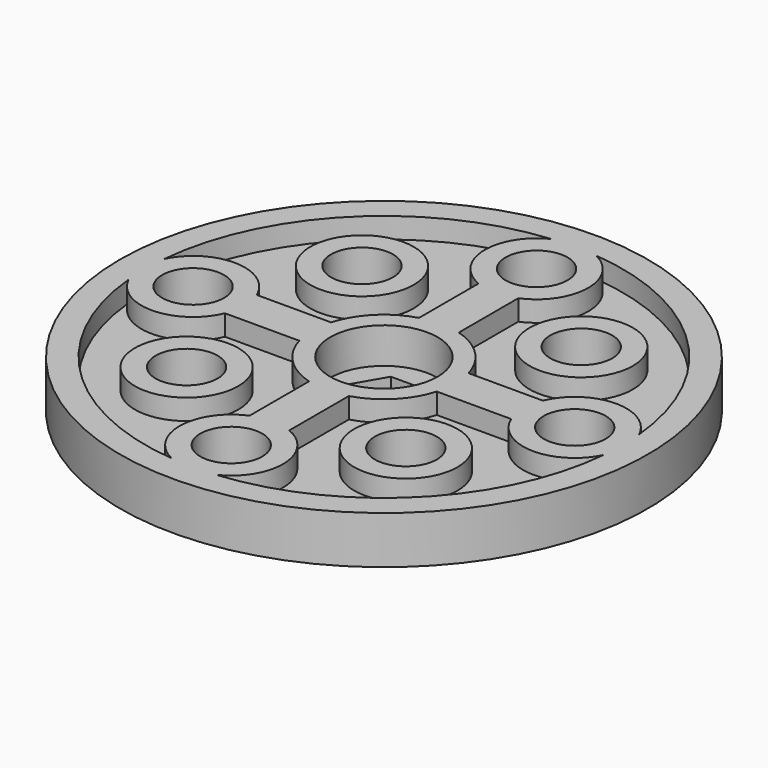
from build123d import *

# Parameters (mm, degrees)
F0_R     = 3.375
F0_R_2   = 1.95
F1_DEPTH = 3
F0_R_3   = 3.25
F2_DEPTH = 1.7
F3_DEPTH = 3
F4_R     = 3.375
F5_DEPTH = 2.25
F6_R     = 4.5310889132
F7_DEPTH = 3.75
F8_R     = 0.75


# Not quite as in the source:
# - a feature names something its author has since deleted; it is built from what else it names


with BuildPart() as f1:
    # F0 (on Top) → F1 (new body)
    with BuildSketch(Plane.XY):
        with BuildLine():
            ThreePointArc((16.6, 0), (0, 16.6), (-16.6, 0))
            ThreePointArc((-16.6, 0), (0, -16.6), (16.6, 0))
        make_face()
        with BuildLine():
            ThreePointArc((14.9348958333, 1.3960252317), (14.9837151184, 0.698771243), (15, 0))
            ThreePointArc((15, 0), (14.9837151184, -0.698771243), (14.9348958333, -1.3960252317))
            ThreePointArc((14.9348958333, -1.3960252317), (10.6066017178, -10.6066017178), (1.3960252317, -14.9348958333))
            ThreePointArc((1.3960252317, -14.9348958333), (0, -15), (-1.3960252317, -14.9348958333))
            ThreePointArc((-1.3960252317, -14.9348958333), (-10.6066017178, -10.6066017178), (-14.9348958333, -1.3960252317))
            ThreePointArc((-14.9348958333, -1.3960252317), (-14.9837151184, -0.698771243), (-15, 0))
            ThreePointArc((-15, 0), (-14.9837151184, 0.698771243), (-14.9348958333, 1.3960252317))
            ThreePointArc((-14.9348958333, 1.3960252317), (-10.6066017178, 10.6066017178), (-1.3960252317, 14.9348958333))
            ThreePointArc((-1.3960252317, 14.9348958333), (0, 15), (1.3960252317, 14.9348958333))
            ThreePointArc((1.3960252317, 14.9348958333), (10.6066017178, 10.6066017178), (14.9348958333, 1.3960252317))
        make_face(mode=Mode.SUBTRACT)
        with BuildLine():
            ThreePointArc((1.25, -4.3229041164), (3.1819805153, -3.1819805153), (4.3229041164, -1.25))
            ThreePointArc((4.3229041164, -1.25), (4.4555060613, -0.6312414261), (4.5, 0))
            ThreePointArc((4.5, 0), (4.4555060613, 0.6312414261), (4.3229041164, 1.25))
            ThreePointArc((4.3229041164, 1.25), (3.1819805153, 3.1819805153), (1.25, 4.3229041164))
            ThreePointArc((1.25, 4.3229041164), (0, 4.5), (-1.25, 4.3229041164))
            ThreePointArc((-1.25, 4.3229041164), (-3.1819805153, 3.1819805153), (-4.3229041164, 1.25))
            ThreePointArc((-4.3229041164, 1.25), (-4.5, 0), (-4.3229041164, -1.25))
            ThreePointArc((-4.3229041164, -1.25), (-3.1819805153, -3.1819805153), (-1.25, -4.3229041164))
            ThreePointArc((-1.25, -4.3229041164), (0, -4.5), (1.25, -4.3229041164))
        make_face()
        Circle(F0_R, mode=Mode.SUBTRACT)
        Circle(F0_R)
        Polygon((-2.25, 0), (-1.125, 1.9485571585), (1.125, 1.9485571585), (2.25, 0), (1.125, -1.9485571585), (-1.125, -1.9485571585), align=None, mode=Mode.SUBTRACT)
        with BuildLine():
            ThreePointArc((14.9348958333, -1.3960252317), (14.9837151184, -0.698771243), (15, 0))
            ThreePointArc((15, 0), (14.9837151184, 0.698771243), (14.9348958333, 1.3960252317))
            ThreePointArc((14.9348958333, 1.3960252317), (11.9200595209, 3.2490167004), (9, 1.25))
            ThreePointArc((9, 1.25), (8.75, 0), (9, -1.25))
            ThreePointArc((9, -1.25), (11.9200595209, -3.2490167004), (14.9348958333, -1.3960252317))
        make_face()
        with Locations((12, 0)):
            Circle(F0_R_2, mode=Mode.SUBTRACT)
        with BuildLine():
            ThreePointArc((1.25, 9), (3.2490167004, 11.9200595209), (1.3960252317, 14.9348958333))
            ThreePointArc((1.3960252317, 14.9348958333), (0, 15), (-1.3960252317, 14.9348958333))
            ThreePointArc((-1.3960252317, 14.9348958333), (-3.2490167004, 11.9200595209), (-1.25, 9))
            ThreePointArc((-1.25, 9), (0, 8.75), (1.25, 9))
        make_face()
        with Locations((0, 12)):
            Circle(F0_R_2, mode=Mode.SUBTRACT)
        with BuildLine():
            ThreePointArc((-1.3960252317, -14.9348958333), (0, -15), (1.3960252317, -14.9348958333))
            ThreePointArc((1.3960252317, -14.9348958333), (3.2490167004, -11.9200595209), (1.25, -9))
            ThreePointArc((1.25, -9), (0, -8.75), (-1.25, -9))
            ThreePointArc((-1.25, -9), (-3.2490167004, -11.9200595209), (-1.3960252317, -14.9348958333))
        make_face()
        with Locations((0, -12)):
            Circle(F0_R_2, mode=Mode.SUBTRACT)
        with BuildLine():
            ThreePointArc((-9, 1.25), (-11.9200595209, 3.2490167004), (-14.9348958333, 1.3960252317))
            ThreePointArc((-14.9348958333, 1.3960252317), (-14.9837151184, 0.698771243), (-15, 0))
            ThreePointArc((-15, 0), (-14.9837151184, -0.698771243), (-14.9348958333, -1.3960252317))
            ThreePointArc((-14.9348958333, -1.3960252317), (-11.9200595209, -3.2490167004), (-9, -1.25))
            ThreePointArc((-9, -1.25), (-8.75, 0), (-9, 1.25))
        make_face()
        with Locations((-12, 0)):
            Circle(F0_R_2, mode=Mode.SUBTRACT)
        with BuildLine():
            ThreePointArc((9, -1.25), (8.75, 0), (9, 1.25))
            Line((9, 1.25), (6, 1.25))
            Line((6, 1.25), (4.3229041164, 1.25))
            ThreePointArc((4.3229041164, 1.25), (4.4555060613, 0.6312414261), (4.5, 0))
            ThreePointArc((4.5, 0), (4.4555060613, -0.6312414261), (4.3229041164, -1.25))
            Line((4.3229041164, -1.25), (9, -1.25))
        make_face()
        with BuildLine():
            Line((1.25, 4.3229041164), (1.25, 9))
            ThreePointArc((1.25, 9), (0, 8.75), (-1.25, 9))
            Line((-1.25, 9), (-1.25, 6))
            Line((-1.25, 6), (-1.25, 4.3229041164))
            ThreePointArc((-1.25, 4.3229041164), (0, 4.5), (1.25, 4.3229041164))
        make_face()
        with BuildLine():
            ThreePointArc((-1.25, -9), (0, -8.75), (1.25, -9))
            Line((1.25, -9), (1.25, -6))
            Line((1.25, -6), (1.25, -4.3229041164))
            ThreePointArc((1.25, -4.3229041164), (0, -4.5), (-1.25, -4.3229041164))
            Line((-1.25, -4.3229041164), (-1.25, -9))
        make_face()
        with BuildLine():
            Line((-4.3229041164, 1.25), (-9, 1.25))
            ThreePointArc((-9, 1.25), (-8.75, 0), (-9, -1.25))
            Line((-9, -1.25), (-6, -1.25))
            Line((-6, -1.25), (-4.3229041164, -1.25))
            ThreePointArc((-4.3229041164, -1.25), (-4.5, 0), (-4.3229041164, 1.25))
        make_face()
    extrude(amount=F1_DEPTH)



with BuildPart() as f1b:
    # F0 (on Top) → F1, piece 2 (new body)
    with BuildSketch(Plane.XY):
        with Locations((6.8942911166, 6.8942911166)):
            Circle(F0_R_3)
        with Locations((6.8942911166, 6.8942911166)):
            Circle(F0_R_2, mode=Mode.SUBTRACT)
    extrude(amount=F1_DEPTH)


with BuildPart() as f1c:
    # F0 (on Top) → F1, piece 3 (new body)
    with BuildSketch(Plane.XY):
        with Locations((-6.8942911166, 6.8942911166)):
            Circle(F0_R_3)
        with Locations((-6.8942911166, 6.8942911166)):
            Circle(F0_R_2, mode=Mode.SUBTRACT)
    extrude(amount=F1_DEPTH)


with BuildPart() as f1d:
    # F0 (on Top) → F1, piece 4 (new body)
    with BuildSketch(Plane.XY):
        with Locations((-6.8942911166, -6.8942911166)):
            Circle(F0_R_3)
        with Locations((-6.8942911166, -6.8942911166)):
            Circle(F0_R_2, mode=Mode.SUBTRACT)
    extrude(amount=F1_DEPTH)


with BuildPart() as f1e:
    # F0 (on Top) → F1, piece 5 (new body)
    with BuildSketch(Plane.XY):
        with Locations((6.8942911166, -6.8942911166)):
            Circle(F0_R_3)
        with Locations((6.8942911166, -6.8942911166)):
            Circle(F0_R_2, mode=Mode.SUBTRACT)
    extrude(amount=F1_DEPTH)


with BuildPart() as f1_1:
    add(f1.part)

    add(f1b.part)  # F2 merges F1b

    add(f1c.part)  # F2 merges F1c

    add(f1d.part)  # F2 merges F1d

    add(f1e.part)  # F2 merges F1e
    # F0 (on Top) → F2 (join)
    with BuildSketch(Plane.XY):
        with BuildLine():
            ThreePointArc((-1.25, 9), (-3.2490167004, 11.9200595209), (-1.3960252317, 14.9348958333))
            ThreePointArc((-1.3960252317, 14.9348958333), (-10.6066017178, 10.6066017178), (-14.9348958333, 1.3960252317))
            ThreePointArc((-14.9348958333, 1.3960252317), (-11.9200595209, 3.2490167004), (-9, 1.25))
            Line((-9, 1.25), (-4.3229041164, 1.25))
            ThreePointArc((-4.3229041164, 1.25), (-3.1819805153, 3.1819805153), (-1.25, 4.3229041164))
            Line((-1.25, 4.3229041164), (-1.25, 6))
            Line((-1.25, 6), (-1.25, 9))
        make_face()
        with Locations((-6.8942911166, 6.8942911166)):
            Circle(F0_R_3, mode=Mode.SUBTRACT)
        with BuildLine():
            ThreePointArc((9, 1.25), (11.9200595209, 3.2490167004), (14.9348958333, 1.3960252317))
            ThreePointArc((14.9348958333, 1.3960252317), (10.6066017178, 10.6066017178), (1.3960252317, 14.9348958333))
            ThreePointArc((1.3960252317, 14.9348958333), (3.2490167004, 11.9200595209), (1.25, 9))
            Line((1.25, 9), (1.25, 4.3229041164))
            ThreePointArc((1.25, 4.3229041164), (3.1819805153, 3.1819805153), (4.3229041164, 1.25))
            Line((4.3229041164, 1.25), (6, 1.25))
            Line((6, 1.25), (9, 1.25))
        make_face()
        with Locations((6.8942911166, 6.8942911166)):
            Circle(F0_R_3, mode=Mode.SUBTRACT)
        with BuildLine():
            ThreePointArc((1.3960252317, -14.9348958333), (10.6066017178, -10.6066017178), (14.9348958333, -1.3960252317))
            ThreePointArc((14.9348958333, -1.3960252317), (11.9200595209, -3.2490167004), (9, -1.25))
            Line((9, -1.25), (4.3229041164, -1.25))
            ThreePointArc((4.3229041164, -1.25), (3.1819805153, -3.1819805153), (1.25, -4.3229041164))
            Line((1.25, -4.3229041164), (1.25, -6))
            Line((1.25, -6), (1.25, -9))
            ThreePointArc((1.25, -9), (3.2490167004, -11.9200595209), (1.3960252317, -14.9348958333))
        make_face()
        with Locations((6.8942911166, -6.8942911166)):
            Circle(F0_R_3, mode=Mode.SUBTRACT)
        with BuildLine():
            ThreePointArc((-14.9348958333, -1.3960252317), (-10.6066017178, -10.6066017178), (-1.3960252317, -14.9348958333))
            ThreePointArc((-1.3960252317, -14.9348958333), (-3.2490167004, -11.9200595209), (-1.25, -9))
            Line((-1.25, -9), (-1.25, -4.3229041164))
            ThreePointArc((-1.25, -4.3229041164), (-3.1819805153, -3.1819805153), (-4.3229041164, -1.25))
            Line((-4.3229041164, -1.25), (-6, -1.25))
            Line((-6, -1.25), (-9, -1.25))
            ThreePointArc((-9, -1.25), (-11.9200595209, -3.2490167004), (-14.9348958333, -1.3960252317))
        make_face()
        with Locations((-6.8942911166, -6.8942911166)):
            Circle(F0_R_3, mode=Mode.SUBTRACT)
        Circle(F0_R)
        Polygon((-2.25, 0), (-1.125, 1.9485571585), (1.125, 1.9485571585), (2.25, 0), (1.125, -1.9485571585), (-1.125, -1.9485571585), align=None, mode=Mode.SUBTRACT)
    extrude(amount=F2_DEPTH)

    # F0 (on Top) → F3 (join)
    with BuildSketch(Plane.XY):
        with BuildLine():
            ThreePointArc((16.6, 0), (0, 16.6), (-16.6, 0))
            ThreePointArc((-16.6, 0), (0, -16.6), (16.6, 0))
        make_face()
        with BuildLine():
            ThreePointArc((14.9348958333, 1.3960252317), (14.9837151184, 0.698771243), (15, 0))
            ThreePointArc((15, 0), (14.9837151184, -0.698771243), (14.9348958333, -1.3960252317))
            ThreePointArc((14.9348958333, -1.3960252317), (10.6066017178, -10.6066017178), (1.3960252317, -14.9348958333))
            ThreePointArc((1.3960252317, -14.9348958333), (0, -15), (-1.3960252317, -14.9348958333))
            ThreePointArc((-1.3960252317, -14.9348958333), (-10.6066017178, -10.6066017178), (-14.9348958333, -1.3960252317))
            ThreePointArc((-14.9348958333, -1.3960252317), (-14.9837151184, -0.698771243), (-15, 0))
            ThreePointArc((-15, 0), (-14.9837151184, 0.698771243), (-14.9348958333, 1.3960252317))
            ThreePointArc((-14.9348958333, 1.3960252317), (-10.6066017178, 10.6066017178), (-1.3960252317, 14.9348958333))
            ThreePointArc((-1.3960252317, 14.9348958333), (0, 15), (1.3960252317, 14.9348958333))
            ThreePointArc((1.3960252317, 14.9348958333), (10.6066017178, 10.6066017178), (14.9348958333, 1.3960252317))
        make_face(mode=Mode.SUBTRACT)
    extrude(amount=F3_DEPTH)

    # F4 (on face) → F5 (cut)
    with BuildSketch(Plane.XY.offset(3)):
        Circle(F4_R)
        Polygon((-1.125, 1.9485571585), (1.125, 1.9485571585), (2.25, 0), (1.125, -1.9485571585), (-1.125, -1.9485571585), (-2.25, 0), align=None, mode=Mode.SUBTRACT)
    extrude(amount=-F5_DEPTH, mode=Mode.SUBTRACT)

    # F6 (on face) → F7 (join)
    with BuildSketch(Plane(origin=(0, 0, 0), x_dir=(1, 0, 0), z_dir=(0, 0, -1))):
        Circle(F6_R)
        Polygon((-3.5, 0), (-1.75, 3.0310889132), (1.75, 3.0310889132), (3.5, 0), (1.75, -3.0310889132), (-1.75, -3.0310889132), align=None, mode=Mode.SUBTRACT)
    extrude(amount=F7_DEPTH)

    # F8
    f8_edges = [f1_1.edges().sort_by_distance(p)[0] for p in [
        (-4.531089, 0, -3.75),
    ]]
    fillet(f8_edges, radius=F8_R)


solid = f1_1.part
